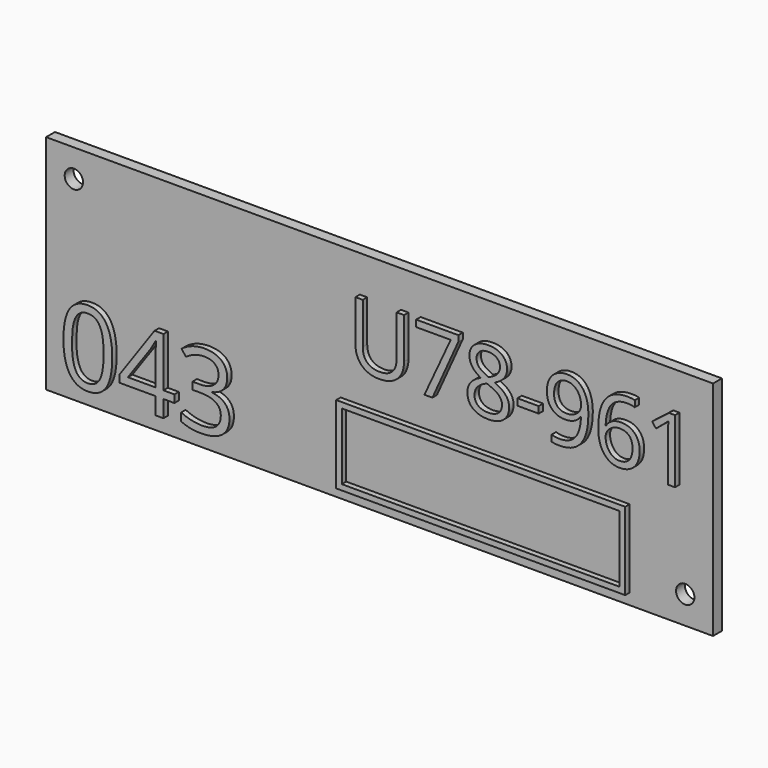
from build123d import *

# Parameters (mm, degrees)
F0_W         = 120
F0_H         = 40
F1_DEPTH     = 2
F3_D         = 3.3
F4_TEXT_SIZE = 15.99800025
F5_DEPTH     = 1
F6_TEXT_SIZE = 18.5894526641
F7_DEPTH     = 1
F8_W         = 52
F8_H         = 14
F8_W_2       = 49.99999962
F8_H_2       = 11.99999962
F9_DEPTH     = 1


# Not quite as in the source:
# - Text() gives the source's letters only with a copy of the font that has no kerning and outlines rounded to 1/6400 em; it was checked with that copy


with BuildPart() as f1:
    # F0 (on Front) → F1 (new body)
    with BuildSketch(Plane.XZ):
        Rectangle(F0_W, F0_H)
    extrude(amount=F1_DEPTH)

    # F3 (through all)
    with Locations(Plane.XZ.offset(2)):
        with Locations((-55, 15), (55, -15)):
            Hole(F3_D / 2)

    # F4 (on face) → F5 (join)
    with BuildSketch(Plane.XZ.offset(2)):
        with Locations((-5, 2)):
            Text('U78-961', F4_TEXT_SIZE, font='Open Sans', text_align=(TextAlign.LEFT, TextAlign.BOTTOM))
    extrude(amount=F5_DEPTH)

    # F6 (on face) → F7 (join)
    with BuildSketch(Plane.XZ.offset(2)):
        with Locations((-57, -17)):
            Text('043', F6_TEXT_SIZE, font='Open Sans', text_align=(TextAlign.LEFT, TextAlign.BOTTOM))
    extrude(amount=F7_DEPTH)

    # F8 (on face) → F9 (join)
    with BuildSketch(Plane.XZ.offset(2)):
        with Locations((19, -11)):
            Rectangle(F8_W, F8_H)
        with Locations((19, -11)):
            Rectangle(F8_W_2, F8_H_2, mode=Mode.SUBTRACT)
    extrude(amount=F9_DEPTH)


solid = f1.part
